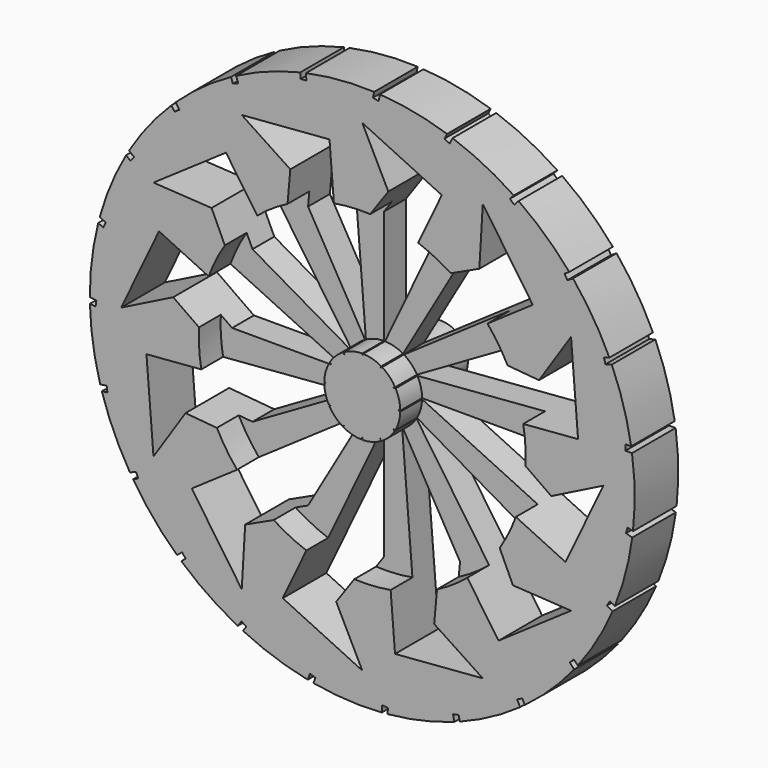
from build123d import *

# Parameters (mm, degrees)
F0_R     = 31.75
F1_DEPTH = 6.35
F3_DEPTH = 6.35
F5_DEPTH = 6.35
F6_R     = 19.05
F6_R_2   = 4.4298133356
F7_DEPTH = 3.175
F8_R     = 3.175
F9_DEPTH = 5.08


with BuildPart() as f1:
    # F0 (on Front) → F1 (new body)
    with BuildSketch(Plane.XZ):
        Circle(F0_R)
    extrude(amount=-F1_DEPTH)

    # F2 (on face) → F3 (cut, through all)
    with BuildSketch(Plane(origin=(0, 6.35, 0), x_dir=(-1, 0, 0), z_dir=(0, 1, 0))):
        with BuildLine():
            Line((-30.6774537772, 5.0991588165), (-31.3378537772, 5.0991588165))
            ThreePointArc((-31.3378537772, 5.0991588165), (-31.3904379038, 4.7647568888), (-31.4394537772, 4.4298133356))
            Line((-31.4394537772, 4.4298133356), (-30.6774537772, 4.4298133356))
            Line((-30.6774537772, 4.4298133356), (-30.6774537772, 5.0991588165))
        make_face()
        with BuildLine():
            Line((-28.1641139896, 13.1867461518), (-28.8000245662, 13.3649199394))
            ThreePointArc((-28.8000245662, 13.3649199394), (-28.940879291, 13.0571055698), (-29.0784442121, 12.7478069566))
            Line((-29.0784442121, 12.7478069566), (-28.3447012391, 12.542221817))
            Line((-28.3447012391, 12.542221817), (-28.1641139896, 13.1867461518))
        make_face()
        with BuildLine():
            Line((-23.5619707096, 20.2963328503), (-24.1262292844, 20.6394660909))
            ThreePointArc((-24.1262292844, 20.6394660909), (-24.344908057, 20.3810684631), (-24.5608194648, 20.120354053))
            Line((-24.5608194648, 20.120354053), (-23.9097518785, 19.7244310831))
            Line((-23.9097518785, 19.7244310831), (-23.5619707096, 20.2963328503))
        make_face()
        with BuildLine():
            Line((-17.2123438509, 25.9006333909), (-17.6631019467, 26.3832774617))
            ThreePointArc((-17.6631019467, 26.3832774617), (-17.9433863629, 26.1934607456), (-18.221631096, 26.0006665338))
            Line((-18.221631096, 26.0006665338), (-17.7015256009, 25.443769529))
            Line((-17.7015256009, 25.443769529), (-17.2123438509, 25.9006333909))
        make_face()
        with BuildLine():
            Line((-9.5861561901, 29.5840024403), (-9.889983141, 30.1703618386))
            ThreePointArc((-9.889983141, 30.1703618386), (-10.2110857878, 30.0632038717), (-10.5310277073, 29.9526285229))
            Line((-10.5310277073, 29.9526285229), (-10.1804581486, 29.2760599864))
            Line((-10.1804581486, 29.2760599864), (-9.5861561901, 29.5840024403))
        make_face()
        with BuildLine():
            Line((-1.2490071783, 31.0732613666), (-1.3833695293, 31.7198484981))
            ThreePointArc((-1.3833695293, 31.7198484981), (-1.7214756924, 31.7032966967), (-2.0593861698, 31.6831410786))
            Line((-2.0593861698, 31.6831410786), (-1.9043526878, 30.9370790037))
            Line((-1.9043526878, 30.9370790037), (-1.2490071783, 31.0732613666))
        make_face()
        with BuildLine():
            Line((7.180774982, 30.2579586481), (7.2258422718, 30.9168191033))
            ThreePointArc((7.2258422718, 30.9168191033), (6.8958083798, 30.9921010386), (6.5649906189, 31.0638600012))
            Line((6.5649906189, 31.0638600012), (6.5129898999, 30.3036363991))
            Line((6.5129898999, 30.3036363991), (7.180774982, 30.2579586481))
        make_face()
        with BuildLine():
            Line((15.0779919118, 27.1985615575), (15.2991464077, 27.8208306705))
            ThreePointArc((15.2991464077, 27.8208306705), (15.0016618908, 27.9823630259), (14.7024720862, 28.1407145352))
            Line((14.7024720862, 28.1407145352), (14.4472938217, 27.4227117126))
            Line((14.4472938217, 27.4227117126), (15.0779919118, 27.1985615575))
        make_face()
        with BuildLine():
            Line((21.8569431587, 22.1219715814), (22.2377828434, 22.6614984988))
            ThreePointArc((22.2377828434, 22.6614984988), (21.9949107673, 22.8973011584), (21.7495384582, 23.1305010074))
            Line((21.7495384582, 23.1305010074), (21.3101080528, 22.5079699489))
            Line((21.3101080528, 22.5079699489), (21.8569431587, 22.1219715814))
        make_face()
        with BuildLine():
            Line((27.0148649204, 15.4046961744), (27.5271446568, 15.8214666528))
            ThreePointArc((27.5271446568, 15.8214666528), (27.3568977323, 16.1140512121), (27.1835410603, 16.4048040349))
            Line((27.1835410603, 16.4048040349), (26.5924490568, 15.9239150213))
            Line((26.5924490568, 15.9239150213), (27.0148649204, 15.4046961744))
        make_face()
        with BuildLine():
            Line((30.1692177357, 7.5449249239), (30.7749440792, 7.8080290036))
            ThreePointArc((30.7749440792, 7.8080290036), (30.6899487419, 8.1356958043), (30.6014647784, 8.462437794))
            Line((30.6014647784, 8.462437794), (29.9025497666, 8.1588561636))
            Line((29.9025497666, 8.1588561636), (30.1692177357, 7.5449249239))
        make_face()
        with BuildLine():
            Line((29.697386948, -9.2289110598), (30.3516359468, -9.3188355148))
            ThreePointArc((30.3516359468, -9.3188355148), (30.4492646919, -8.994708429), (30.5434321701, -8.6695588854))
            Line((30.5434321701, -8.6695588854), (29.7885294793, -8.5657998988))
            Line((29.7885294793, -8.5657998988), (29.697386948, -9.2289110598))
        make_face()
        with BuildLine():
            ThreePointArc((31.7403066853, -0.7844944374), (31.7468666505, -0.4460469429), (31.7498178462, -0.1075487449))
            Line((31.7498178462, -0.1075487449), (30.9949151553, -0.2113077315))
            Line((30.9949151553, -0.2113077315), (31.0860576866, -0.8744188925))
            Line((31.0860576866, -0.8744188925), (31.7403066853, -0.7844944374))
        make_face()
        with BuildLine():
            Line((26.1061968761, -16.8989371132), (26.7119232196, -17.162041193))
            ThreePointArc((26.7119232196, -17.162041193), (26.8933800672, -16.8762735389), (27.0717798569, -16.588587504))
            Line((27.0717798569, -16.588587504), (26.3728648452, -16.2850058735))
            Line((26.3728648452, -16.2850058735), (26.1061968761, -16.8989371132))
        make_face()
        with BuildLine():
            Line((20.5788296098, -23.3156463085), (21.0911093462, -23.7324167869))
            ThreePointArc((21.0911093462, -23.7324167869), (21.342936472, -23.5062026443), (21.5923374769, -23.2773164752))
            Line((21.5923374769, -23.2773164752), (21.0012454734, -22.7964274616))
            Line((21.0012454734, -22.7964274616), (20.5788296098, -23.3156463085))
        make_face()
        with BuildLine():
            Line((13.5252246932, -28.003140679), (13.9060643779, -28.5426675964))
            ThreePointArc((13.9060643779, -28.5426675964), (14.2095849161, -28.3927842332), (14.5114902045, -28.23967337))
            Line((14.5114902045, -28.23967337), (14.0720597991, -27.6171423115))
            Line((14.0720597991, -27.6171423115), (13.5252246932, -28.003140679))
        make_face()
        with BuildLine():
            Line((5.4685157349, -30.6137702113), (5.6896702307, -31.2360393242))
            ThreePointArc((5.6896702307, -31.2360393242), (6.0223734514, -31.1736029039), (6.3543920894, -31.1076228789))
            Line((6.3543920894, -31.1076228789), (6.0992138249, -30.3896200562))
            Line((6.0992138249, -30.3896200562), (5.4685157349, -30.6137702113))
        make_face()
        with BuildLine():
            Line((-2.9937680187, -30.9539164556), (-2.9487007289, -31.6127769108))
            ThreePointArc((-2.9487007289, -31.6127769108), (-2.6114899016, -31.642418057), (-2.2739822177, -31.6684623067))
            Line((-2.2739822177, -31.6684623067), (-2.3259829366, -30.9082387046))
            Line((-2.3259829366, -30.9082387046), (-2.9937680187, -30.9539164556))
        make_face()
        with BuildLine():
            Line((-11.2340176939, -28.9983523212), (-11.3683800449, -29.6449394527))
            ThreePointArc((-11.3683800449, -29.6449394527), (-11.0516709953, -29.7644598172), (-10.7337056664, -29.8805967589))
            Line((-10.7337056664, -29.8805967589), (-10.5786721844, -29.1345346841))
            Line((-10.5786721844, -29.1345346841), (-11.2340176939, -28.9983523212))
        make_face()
        with BuildLine():
            Line((-18.641091669, -24.8921130537), (-18.9449186199, -25.478472452))
            ThreePointArc((-18.9449186199, -25.478472452), (-18.6722002094, -25.6790077561), (-18.3973592692, -25.8766240441))
            Line((-18.3973592692, -25.8766240441), (-18.0467897105, -25.2000555077))
            Line((-18.0467897105, -25.2000555077), (-18.641091669, -24.8921130537))
        make_face()
        with BuildLine():
            Line((-24.6656411523, -18.9397396349), (-25.116399248, -19.4223837057))
            ThreePointArc((-25.116399248, -19.4223837057), (-24.9078977536, -19.6890611634), (-24.6965648974, -19.9535005016))
            Line((-24.6965648974, -19.9535005016), (-24.1764594023, -19.3966034968))
            Line((-24.1764594023, -19.3966034968), (-24.6656411523, -18.9397396349))
        make_face()
        with BuildLine():
            Line((-28.8608528691, -11.5826923709), (-29.4251114439, -11.9258256115))
            ThreePointArc((-29.4251114439, -11.9258256115), (-29.2962904674, -12.2388669757), (-29.1641392865, -12.5505171081))
            Line((-29.1641392865, -12.5505171081), (-28.5130717002, -12.1545941381))
            Line((-28.5130717002, -12.1545941381), (-28.8608528691, -11.5826923709))
        make_face()
        with BuildLine():
            Line((-30.9155871582, -3.3666098011), (-31.5514977348, -3.5447835888))
            ThreePointArc((-31.5514977348, -3.5447835888), (-31.5119113389, -3.8809720135), (-31.4687428817, -4.2167192755))
            Line((-31.4687428817, -4.2167192755), (-30.7349999087, -4.0111341358))
            Line((-30.7349999087, -4.0111341358), (-30.9155871582, -3.3666098011))
        make_face()
    extrude(amount=-F3_DEPTH, mode=Mode.SUBTRACT)

    # F4 (on face) → F5 (cut, through all)
    with BuildSketch(Plane.XZ):
        Polygon((-23.6905380548, 9.2680157343), (-28.0955714155, 0), (-22.0300974054, 3.0369036725), (-17.7069714155, 0), (-4.191, 0), align=None)
        Polygon((-17.5601721646, 13.6450844319), (-15.3346870699, 8.8534857078), (-3.6295124673, 2.0955), (-15.8825999176, 19.8716060959), (-24.3314785797, 14.0477857078), align=None)
        Polygon((-8.3850129735, 20.5970758371), (-8.8534857078, 15.3346870699), (-2.0955, 3.6295124673), (-3.8189319588, 25.1506156519), (-14.0477857078, 24.3314785797), align=None)
        Polygon((3.0369036725, 22.0300974054), (0, 17.7069714155), (0, 4.191), (9.2680157343, 23.6905380548), (0, 28.0955714155), align=None)
        Polygon((13.6450844319, 17.5601721646), (8.8534857078, 15.3346870699), (2.0955, 3.6295124673), (19.8716060959, 15.8825999176), (14.0477857078, 24.3314785797), align=None)
        Polygon((20.5970758371, 8.3850129735), (15.3346870699, 8.8534857078), (3.6295124673, 2.0955), (25.1506156519, 3.8189319588), (24.3314785797, 14.0477857078), align=None)
        Polygon((22.0300974054, -3.0369036725), (17.7069714155, 0), (4.191, 0), (23.6905380548, -9.2680157343), (28.0955714155, 0), align=None)
        Polygon((17.5601721646, -13.6450844319), (15.3346870699, -8.8534857078), (3.6295124673, -2.0955), (15.8825999176, -19.8716060959), (24.3314785797, -14.0477857078), align=None)
        Polygon((8.3850129735, -20.5970758371), (8.8534857078, -15.3346870699), (2.0955, -3.6295124673), (3.8189319588, -25.1506156519), (14.0477857078, -24.3314785797), align=None)
        Polygon((-3.0369036725, -22.0300974054), (0, -17.7069714155), (0, -4.191), (-9.2680157343, -23.6905380548), (0, -28.0955714155), align=None)
        Polygon((-13.6450844319, -17.5601721646), (-8.8534857078, -15.3346870699), (-2.0955, -3.6295124673), (-19.8716060959, -15.8825999176), (-14.0477857078, -24.3314785797), align=None)
        Polygon((-20.5970758371, -8.3850129735), (-15.3346870699, -8.8534857078), (-3.6295124673, -2.0955), (-25.1506156519, -3.8189319588), (-24.3314785797, -14.0477857078), align=None)
    extrude(amount=-F5_DEPTH, mode=Mode.SUBTRACT)

    # F6 (on face) → F7 (cut)
    with BuildSketch(Plane.XZ):
        Circle(F6_R)
        Circle(F6_R_2, mode=Mode.SUBTRACT)
    extrude(amount=-F7_DEPTH, mode=Mode.SUBTRACT)

    # F8 (on face) → F9 (join)
    with BuildSketch(Plane(origin=(0, 6.35, 0), x_dir=(-1, 0, 0), z_dir=(0, 1, 0))):
        Circle(F8_R)
    extrude(amount=F9_DEPTH)


solid = f1.part
